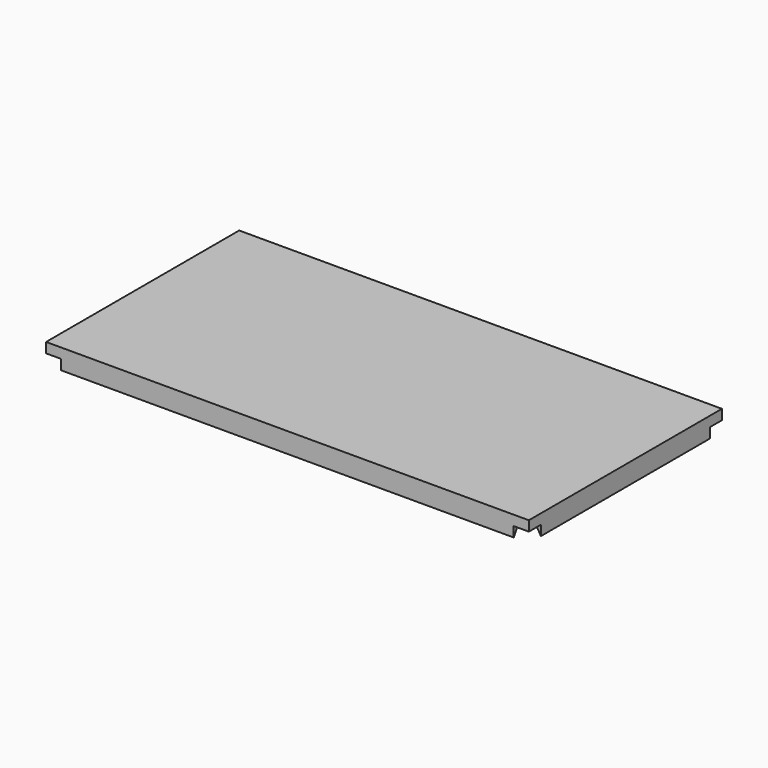
from build123d import *

# Parameters (mm, degrees)
F0_W     = 2438.4
F0_H     = 1219.2
F1_DEPTH = 50.8
F3_DEPTH = 1143
F6_DEPTH = 533.4


# Not quite as in the source:
# - a pattern or mirror of a feature is missing from the dataset's text; its kind, count and spacing are read off the source's solid


with BuildPart() as f1:
    # F0 (on Top) → F1 (new body)
    with BuildSketch(Plane.XY):
        Rectangle(F0_W, F0_H)
    extrude(amount=F1_DEPTH)

    # F2 (on Right) → F3 (join, symmetric)
    with BuildSketch(Plane.YZ):
        Polygon((-609.6, -50.8), (-580.2706063252, 0), (-609.6, 0), align=None)
    f3 = extrude(amount=F3_DEPTH, both=True)

    # F3_copies: F3 across plane
    add(f3.mirror(Plane.ZX))

    # F5 (on Front) → F6 (join, symmetric)
    with BuildSketch(Plane.XZ):
        Polygon((1219.2, 0), (1189.8706063252, 0), (1219.2, -50.8), align=None)
    f6 = extrude(amount=F6_DEPTH, both=True)

    # F6_copies: F6 across plane
    add(f6.mirror(Plane(origin=(0, 0, 0), x_dir=(0, 0, -1), z_dir=(-1, 0, 0))))


solid = f1.part
